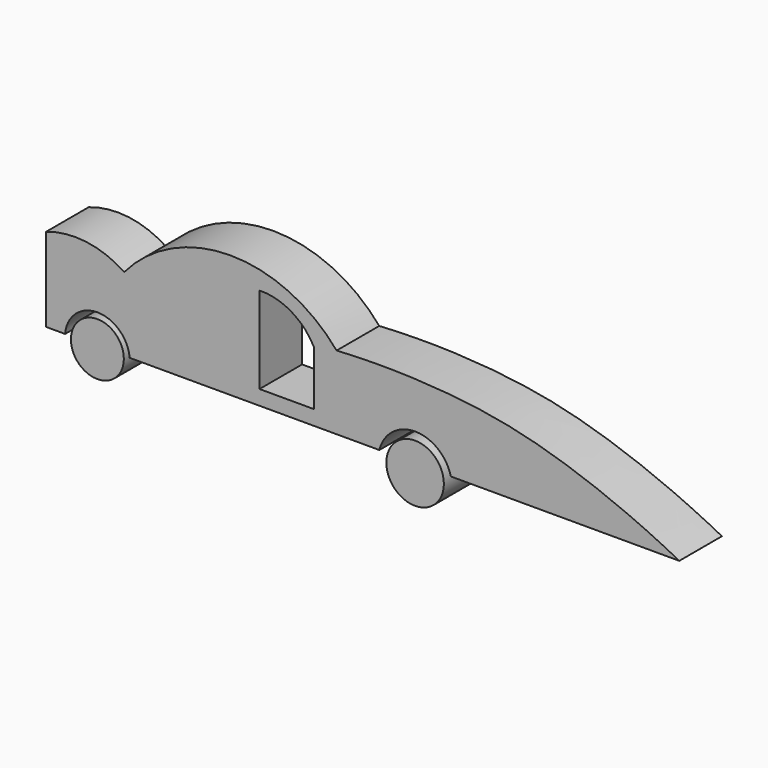
from build123d import *

# Parameters (mm, degrees)
F0_R     = 13.7110734448
F1_DEPTH = 25.4
F0_R_2   = 12.6105017718


# Not quite as in the source:
# - a feature of the source that left no trace in its solid (it failed there, or was rolled back) is left out


with BuildPart() as f1:
    # F0 (on Front) → F1 (new body)
    with BuildSketch(Plane.XZ):
        with Locations((-33.0394776538, -15.1831200019)):
            Circle(F0_R)
    extrude(amount=F1_DEPTH)


with BuildPart() as f1b:
    # F0 (on Front) → F1, piece 2 (new body)
    with BuildSketch(Plane.XZ):
        with BuildLine():
            Line((92.9161560608, -10.9940236434), (92.9169878364, -10.9940236434))
            add(Edge.make_bspline(
                [(-70.4575031996, 24.1402760148), (-70.4399876122, 24.0586483776), (15.7471046571, 31.0948765027), (92.9262256442, -11.0533031958), (92.9169878364, -10.9940236434)],
                knots=[0.5000562346, 0.5000562346, 0.5000562346, 0.5000562346, 0.7490092067, 1, 1, 1, 1], degree=3))
            ThreePointArc((-70.4575031996, 24.1402760148), (-121.0832968354, 47.6414032219), (-171.7090904713, 24.1402760148))
            ThreePointArc((-171.7090904713, 24.1402760148), (-189.7700354442, 30.9387637162), (-208.9654356241, 28.9503522217))
            Line((-208.9654356241, 28.9503522217), (-208.9654356241, -10.9940236434))
            Line((-208.9654356241, -10.9940236434), (-199.9072730541, -10.9940236434))
            ThreePointArc((-199.9072730541, -10.9940236434), (-184.5083907247, 3.107127368), (-169.1095083952, -10.9940236434))
            Line((-169.1095083952, -10.9940236434), (-154.7798216343, -10.9940236434))
            Line((-154.7798216343, -10.9940236434), (-50.079613924, -10.9940236434))
            ThreePointArc((-50.079613924, -10.9940236434), (-33.0394776538, 2.3643804585), (-15.9993413836, -10.9940236434))
            Line((-15.9993413836, -10.9940236434), (92.9161560608, -10.9940236434))
        make_face()
        with BuildLine():
            ThreePointArc((-107.2120293975, 37.4046415091), (-92.0155707574, 33.43707411), (-81.2452882528, 22.0057591796))
            Line((-81.2452882528, 22.0057591796), (-81.2452882528, -3.9609856904))
            Line((-81.2452882528, -3.9609856904), (-107.2120293975, -3.9609856904))
            Line((-107.2120293975, -3.9609856904), (-107.2120293975, 37.4046415091))
        make_face(mode=Mode.SUBTRACT)
    extrude(amount=F1_DEPTH)


with BuildPart() as f1c:
    # F0 (on Front) → F1, piece 3 (new body)
    with BuildSketch(Plane.XZ):
        with Locations((-184.5083907247, -12.3514701781)):
            Circle(F0_R_2)
    extrude(amount=F1_DEPTH)


solid = Compound([f1.part, f1b.part, f1c.part])
